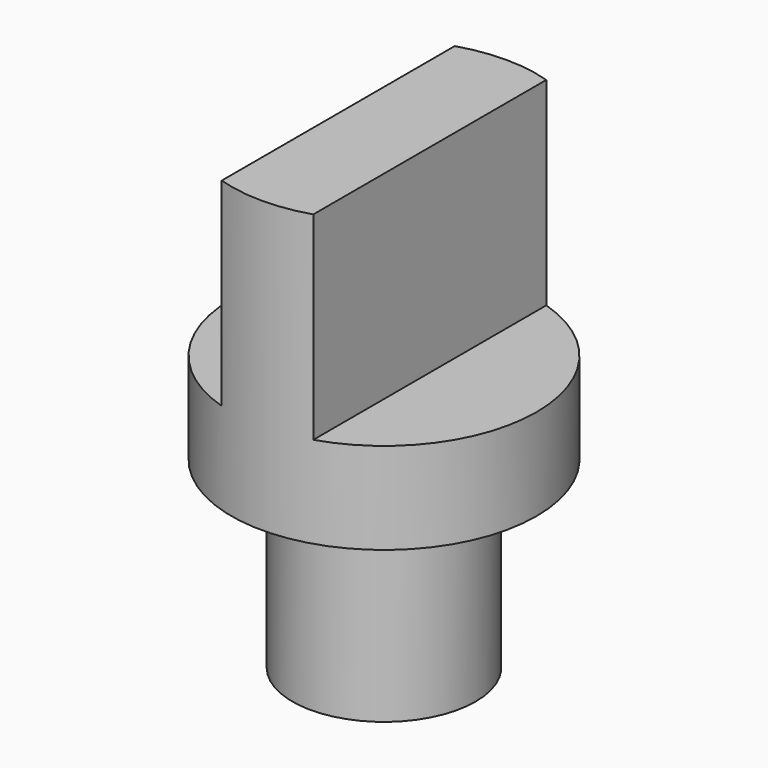
from build123d import *

# Parameters (mm, degrees)
F0_R     = 10
F1_DEPTH = 31
F3_DEPTH = 13
F4_R     = 10
F4_R_2   = 6
F5_DEPTH = 12


with BuildPart() as f1:
    # F0 (on Top) → F1 (new body)
    with BuildSketch(Plane.XY):
        Circle(F0_R)
    extrude(amount=F1_DEPTH)

    # F2 (on face) → F3 (cut)
    with BuildSketch(Plane.XY.offset(31)):
        with BuildLine():
            Line((3, 9.5393920142), (3, 0))
            Line((3, 0), (3, -9.5393920142))
            ThreePointArc((3, -9.5393920142), (8.0622577483, -5.9160797831), (10, 0))
            ThreePointArc((10, 0), (8.0622577483, 5.9160797831), (3, 9.5393920142))
        make_face()
        with BuildLine():
            Line((-3, -9.5393920142), (-3, 0))
            Line((-3, 0), (-3, 9.5393920142))
            ThreePointArc((-3, 9.5393920142), (-10, 0), (-3, -9.5393920142))
        make_face()
    extrude(amount=-F3_DEPTH, mode=Mode.SUBTRACT)

    # F4 (on face) → F5 (cut)
    with BuildSketch(Plane(origin=(0, 0, 0), x_dir=(1, 0, 0), z_dir=(0, 0, -1))):
        Circle(F4_R)
        Circle(F4_R_2, mode=Mode.SUBTRACT)
    extrude(amount=-F5_DEPTH, mode=Mode.SUBTRACT)


solid = f1.part
